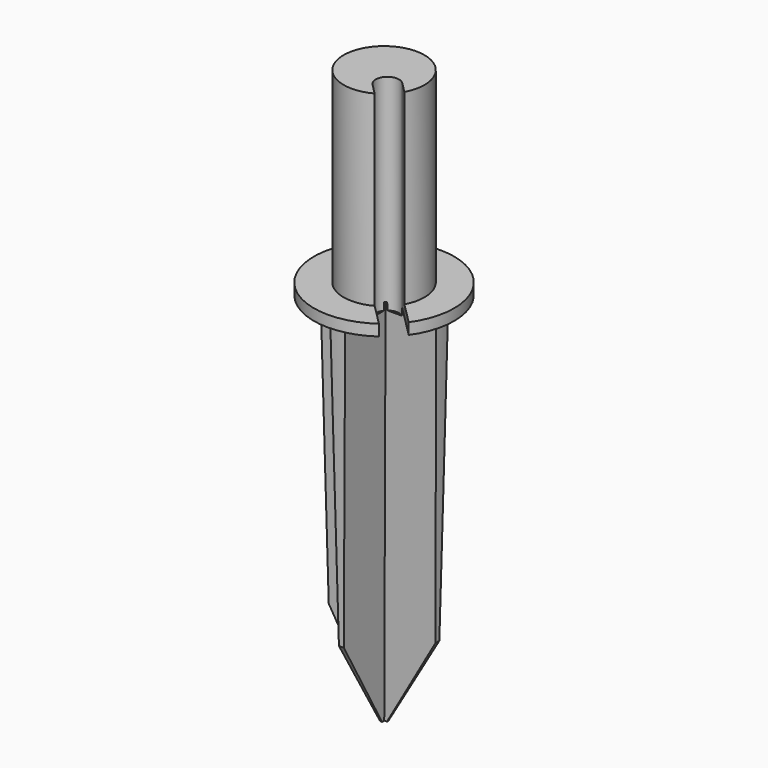
from build123d import *

# Parameters (mm, degrees)
F0_R                   = 19.05
F1_DEPTH               = 3.048
F2_R                   = 10.9855
F3_DEPTH               = 50.8
F5_DEPTH               = 101.6
DRAFT_F5_DRAFTED_ANGLE = 1
F6_R                   = 38.1
F6_R_2                 = 1.016
F7_DEPTH               = 25.4
F7_TAPER               = 30
F9_DEPTH               = 55.88


# Not quite as in the source:
# - an extrude with a draft is written as a straight extrude whose walls are then drafted


with BuildPart() as f1:
    # F0 (on Top) → F1 (new body)
    with BuildSketch(Plane.XY):
        Circle(F0_R)
    extrude(amount=F1_DEPTH)

    # F2 (on face) → F3 (join)
    with BuildSketch(Plane.XY.offset(3.048)):
        Circle(F2_R)
    extrude(amount=F3_DEPTH)


with BuildPart() as f5_drafted:
    # F4 (on face) → F5 (new body)
    with BuildSketch(Plane(origin=(0, 0, 0), x_dir=(1, 0, 0), z_dir=(0, 0, -1))):
        with BuildLine():
            Line((2.032, -2.032), (15.7444149145, -2.032))
            ThreePointArc((15.7444149145, -2.032), (15.875, 0), (15.7444149145, 2.032))
            Line((15.7444149145, 2.032), (2.032, 2.032))
            Line((2.032, 2.032), (2.032, 15.7444149145))
            ThreePointArc((2.032, 15.7444149145), (0, 15.875), (-2.032, 15.7444149145))
            Line((-2.032, 15.7444149145), (-2.032, 2.032))
            Line((-2.032, 2.032), (-15.7444149145, 2.032))
            ThreePointArc((-15.7444149145, 2.032), (-15.875, 0), (-15.7444149145, -2.032))
            Line((-15.7444149145, -2.032), (-2.032, -2.032))
            Line((-2.032, -2.032), (-2.032, -15.7444149145))
            ThreePointArc((-2.032, -15.7444149145), (0, -15.875), (2.032, -15.7444149145))
            Line((2.032, -15.7444149145), (2.032, -2.032))
        make_face()
    extrude(amount=F5_DEPTH)

    # draft_F5_drafted
    draft_f5_drafted_walls = [f5_drafted.faces().sort_by_distance(p)[0] for p in [
        (2.032, 8.8882074573, -67.7333333333),
        (8.8882074573, 2.032, -67.7333333333),
        (15.875, 0, -67.7333333333),
        (8.8882074573, -2.032, -67.7333333333),
        (2.032, -8.8882074573, -67.7333333333),
        (0, -15.875, -67.7333333333),
        (-2.032, -8.8882074573, -67.7333333333),
        (-8.8882074573, -2.032, -67.7333333333),
        (-15.875, 0, -67.7333333333),
        (-8.8882074573, 2.032, -67.7333333333),
        (-2.032, 8.8882074573, -67.7333333333),
        (0, 15.875, -67.7333333333),
    ]]
    draft(draft_f5_drafted_walls, neutral_plane=Plane(origin=(0, 0, 0), x_dir=(1, 0, 0), z_dir=(0, 0, -1)), angle=DRAFT_F5_DRAFTED_ANGLE)


with BuildPart() as f1_1:
    add(f1.part)

    # join_F5_drafted: union F5_drafted
    add(f5_drafted.part)

    # F6 (on face) → F7 (cut)
    with BuildSketch(Plane(origin=(0, 0, -101.6), x_dir=(1, 0, 0), z_dir=(0, 0, -1))):
        Circle(F6_R)
        Circle(F6_R_2, mode=Mode.SUBTRACT)
    extrude(amount=-F7_DEPTH, taper=F7_TAPER, mode=Mode.SUBTRACT)

    # F8 (on face) → F9 (cut)
    with BuildSketch(Plane.XY.offset(53.848)):
        with BuildLine():
            Line((9.6814806825, -5.1913526219), (6.7351920908, -2.2450640303))
            ThreePointArc((6.7351920908, -2.2450640303), (2.2450640303, -2.2450640303), (2.2450640303, -6.7351920908))
            Line((2.2450640303, -6.7351920908), (5.1913526219, -9.6814806825))
            ThreePointArc((5.1913526219, -9.6814806825), (7.7679215447, -7.7679215447), (9.6814806825, -5.1913526219))
        make_face()
        with BuildLine():
            Line((15.5270419515, -11.036913891), (9.6814806825, -5.1913526219))
            ThreePointArc((9.6814806825, -5.1913526219), (7.7679215447, -7.7679215447), (5.1913526219, -9.6814806825))
            Line((5.1913526219, -9.6814806825), (11.036913891, -15.5270419515))
            ThreePointArc((11.036913891, -15.5270419515), (13.4703841816, -13.4703841816), (15.5270419515, -11.036913891))
        make_face()
    extrude(amount=-F9_DEPTH, mode=Mode.SUBTRACT)


solid = f1_1.part
